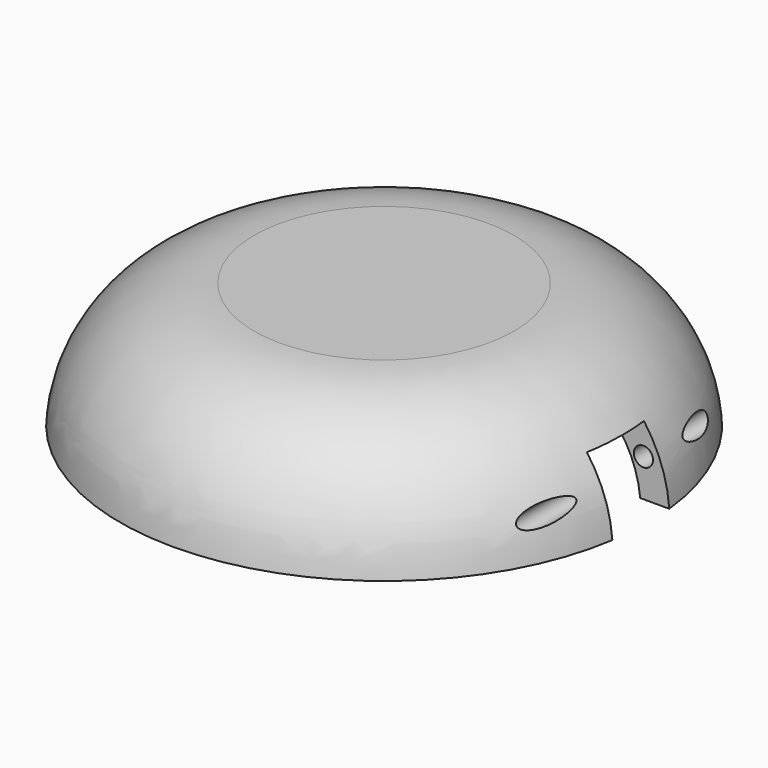
from build123d import *

# Parameters (mm, degrees)
F0_R          = 34.925
F1_DEPTH      = 16.51
F3_T          = -3.81
F4_W          = 11.3246641613
F4_H          = 9.144
F5_DEPTH      = 9.144
F6_R          = 1.27
F7_DEPTH      = 25.4
F7_DEPTH_BACK = 25.4


# Not quite as in the source:
# - a fillet or chamfer that OpenCascade refuses, or shapes differently, is made with other operations: its cross-section is extruded or revolved along the edge and cut away or added


with BuildPart() as f1:
    # F0 (on Top) → F1 (new body)
    with BuildSketch(Plane.XY):
        Circle(F0_R)
    extrude(amount=F1_DEPTH)

    # F2: fillet of radius 17.78 on 1 edges, made by hand

    # F2_s1 → F2_t2 (revolve, cut)
    with BuildSketch(Plane.XZ):
        with BuildLine():
            ThreePointArc((34.925, 0), (29.3054430024, 11.7436274728), (17.1904151444, 16.51))
            Line((17.1904151444, 16.51), (34.925, 16.51))
            Line((34.925, 16.51), (34.925, 0))
        make_face()
    revolve(axis=Axis((0, 0, 16.51), (0, 0, 1)), mode=Mode.SUBTRACT)

    # F3
    f3_openings = [f1.faces().sort_by_distance(p)[0] for p in [
        (0, 0, 0),
    ]]
    offset(amount=F3_T, openings=f3_openings)

    # F4 (on Top) → F5 (cut)
    with BuildSketch(Plane.XY):
        with Locations((32.6112154871, -0.8110651979)):
            Rectangle(F4_W, F4_H)
    extrude(amount=F5_DEPTH, mode=Mode.SUBTRACT)

    # F6 (on face) → F7 (cut, two sides)
    with BuildSketch(Plane(origin=(0, -5.3830651979, 0), x_dir=(-1, 0, 0), z_dir=(0, 1, 0))) as f7_sk:
        with Locations((-31.2978422578, 4.977144105)):
            Circle(F6_R)
    extrude(amount=-F7_DEPTH, mode=Mode.SUBTRACT)
    extrude(f7_sk.sketch, amount=F7_DEPTH_BACK, mode=Mode.SUBTRACT)


solid = f1.part
